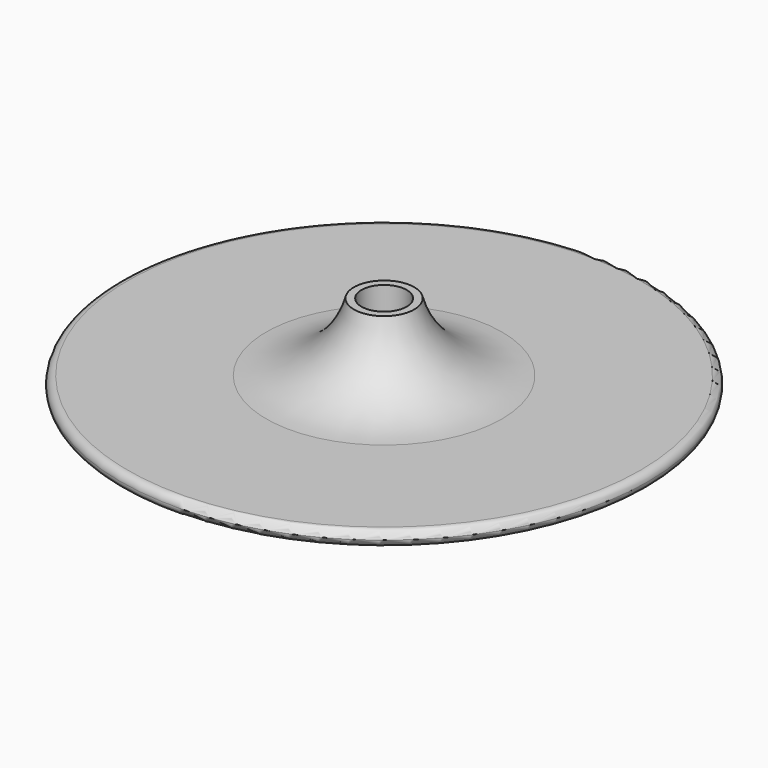
from build123d import *

# Parameters (mm, degrees)
F0_R      = 4
F1_DEPTH  = 10
F2_R      = 35
F3_DEPTH  = 1
F6_R      = 0.99999
F7_R      = 3
F8_DEPTH  = 10.001
F9_R      = 3
F10_DEPTH = 10.001


# Not quite as in the source:
# - a fillet or chamfer that OpenCascade refuses, or shapes differently, is made with other operations: its cross-section is extruded or revolved along the edge and cut away or added
# - a fillet or chamfer is up to 0.001 mm smaller than in the source, because OpenCascade refuses the exact size


with BuildPart() as f1:
    # F0 (on Top) → F1 (new body, symmetric)
    with BuildSketch(Plane.XY):
        Circle(F0_R)
    extrude(amount=F1_DEPTH, both=True)

    # F2 (on Top) → F3 (join, symmetric)
    with BuildSketch(Plane.XY):
        Circle(F2_R)
    extrude(amount=F3_DEPTH, both=True)

    # F4: fillet of radius 12 on 1 edges, made by hand

    # F4_s1 → F4_t2 (revolve)
    with BuildSketch(Plane.XZ):
        with BuildLine():
            ThreePointArc((15.6189500386, 1), (8.2704808103, 3.5131670195), (4, 10))
            Line((4, 10), (4, 1))
            Line((4, 1), (15.6189500386, 1))
        make_face()
    revolve(axis=Axis((0, 0, 1), (0, 0, 1)))

    # F5: fillet of radius 12 on 1 edges, made by hand

    # F5_s1 → F5_t2 (revolve)
    with BuildSketch(Plane.XZ):
        with BuildLine():
            ThreePointArc((4, -10), (8.2704808103, -3.5131670195), (15.6189500386, -1))
            Line((15.6189500386, -1), (4, -1))
            Line((4, -1), (4, -10))
        make_face()
    revolve(axis=Axis((0, 0, -1), (0, 0, 1)))

    # F6 (radius 1 in the source; OpenCascade refuses exactly that, so slightly less here)
    f6_edges = [f1.edges().sort_by_distance(p)[0] for p in [
        (-35, 0, 1),
        (-35, 0, -1),
    ]]
    fillet(f6_edges, radius=F6_R)

    # F7 (on Top) → F8 (cut, through all)
    with BuildSketch(Plane.XY):
        Circle(F7_R)
    extrude(amount=-F8_DEPTH, mode=Mode.SUBTRACT)

    # F9 (on Top) → F10 (cut, through all)
    with BuildSketch(Plane.XY):
        Circle(F9_R)
    extrude(amount=F10_DEPTH, mode=Mode.SUBTRACT)


solid = f1.part
